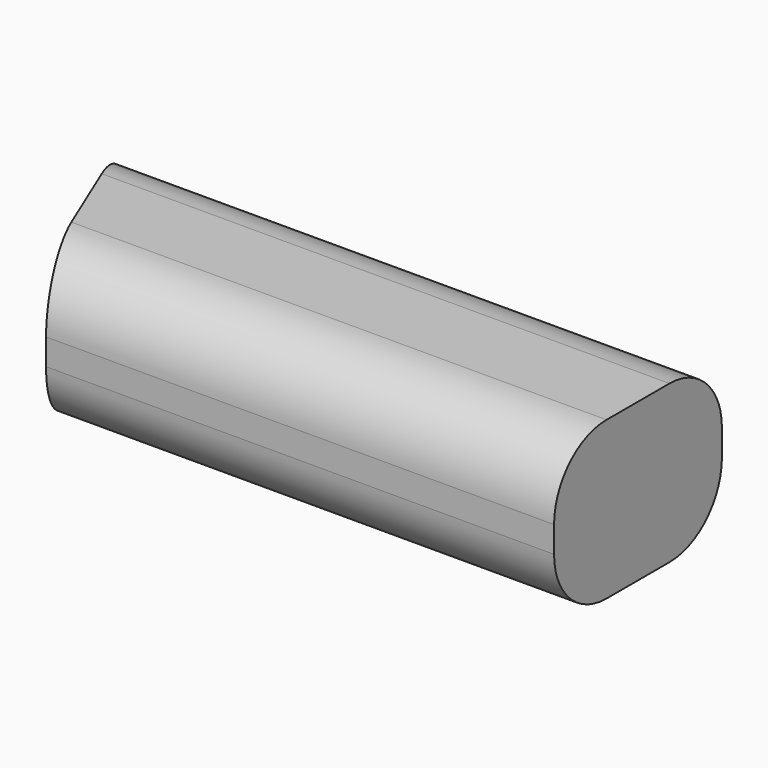
from build123d import *

# Parameters (mm, degrees)
F1_DEPTH = 76.2
F2_R     = 31.75


# Not quite as in the source:
# - a feature names something its author has since deleted; it is built from what else it names


with BuildPart() as f1:
    # F0 (on Top) → F1 (new body)
    with BuildSketch(Plane.XY):
        Polygon((-42.0840979371, 101.6), (0, 0), (246.0318041258, 0), (246.0318041258, 101.6), align=None)
    extrude(amount=F1_DEPTH)

    # F2
    f2_edges = [f1.edges().sort_by_distance(p)[0] for p in [
        (123.015902, 0, 76.2),
        (123.015902, 0, 0),
        (101.973853, 101.6, 76.2),
        (101.973853, 101.6, 0),
    ]]
    fillet(f2_edges, radius=F2_R)


solid = f1.part
